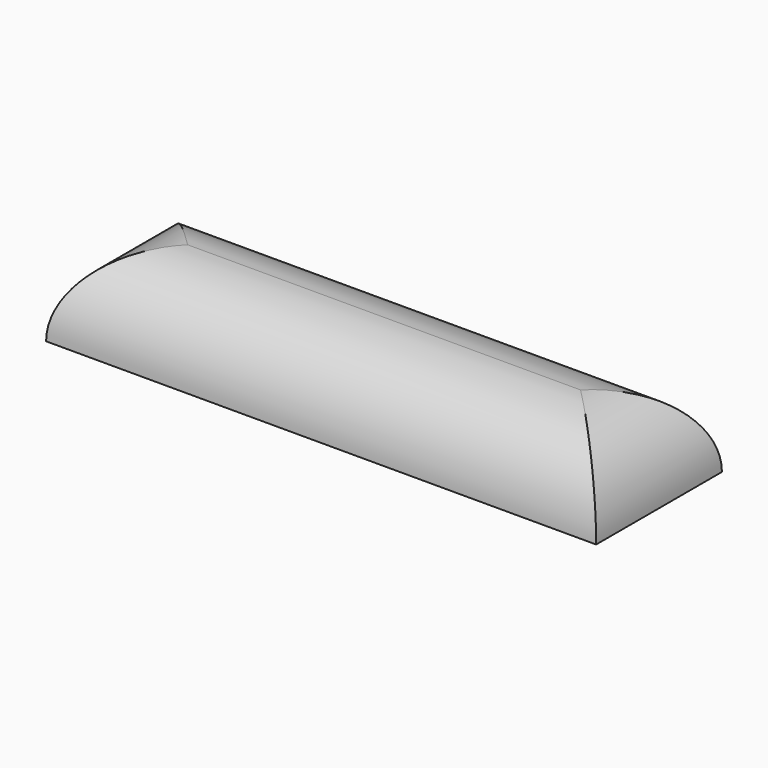
from build123d import *

# Parameters (mm, degrees)
F0_W     = 355.6
F0_H     = 101.6
F1_DEPTH = 50.8
F2_R     = 50.79999


# Not quite as in the source:
# - a fillet or chamfer is up to 0.001 mm smaller than in the source, because OpenCascade refuses the exact size


with BuildPart() as f1:
    # F0 (on Top) → F1 (new body)
    with BuildSketch(Plane.XY):
        Rectangle(F0_W, F0_H)
    extrude(amount=F1_DEPTH)

    # F2 (radius 50.8 in the source; OpenCascade refuses exactly that, so slightly less here)
    f2_edges = [f1.edges().sort_by_distance(p)[0] for p in [
        (0, 50.8, 50.8),
        (0, -50.8, 50.8),
        (177.8, 0, 50.8),
        (-177.8, 0, 50.8),
    ]]
    fillet(f2_edges, radius=F2_R)


solid = f1.part
